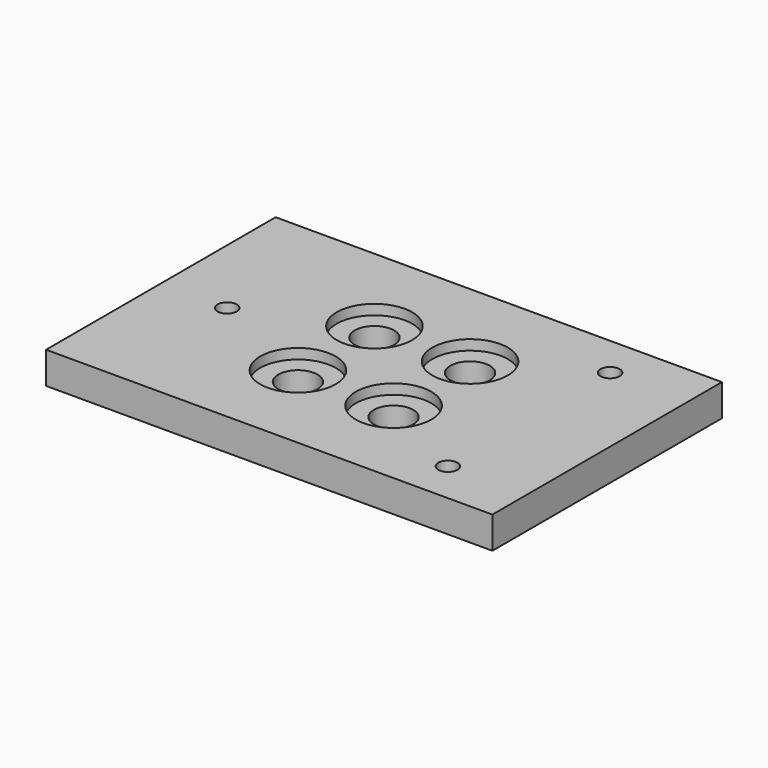
from build123d import *

# Parameters (mm, degrees)
F1_W     = 70
F1_H     = 45
F2_DEPTH = 5
F3_R     = 1.508
F4_DEPTH = 25
F5_R     = 3.0876875
F6_DEPTH = 25
F7_R     = 5.921375
F8_DEPTH = 1.5875


# Not quite as in the source:
# - a length typed as a fraction of an inch, garbled in the dataset ("3 / 203.2 mm" for 3/8 in), is restored


with BuildPart() as f2:
    # F1 (on Top) → F2 (new body)
    with BuildSketch(Plane.XY):
        with Locations((-0.7, 0)):
            Rectangle(F1_W, F1_H)
    extrude(amount=-F2_DEPTH)

    # F3 (on Top) → F4 (cut)
    with BuildSketch(Plane.XY):
        with Locations((-25.3, 0)):
            Circle(F3_R)
        with Locations((22.04, 15.9)):
            Circle(F3_R)
        with Locations((22.04, -15.9)):
            Circle(F3_R)
    extrude(amount=-F4_DEPTH, mode=Mode.SUBTRACT)

    # F5 (on Top) → F6 (cut)
    with BuildSketch(Plane.XY):
        with Locations((-8.2, 7.5)):
            Circle(F5_R)
        with Locations((6.8, 7.5)):
            Circle(F5_R)
        with Locations((-8.2, -7.5)):
            Circle(F5_R)
        with Locations((6.8, -7.5)):
            Circle(F5_R)
    extrude(amount=-F6_DEPTH, mode=Mode.SUBTRACT)

    # F7 (on face) → F8 (cut)
    with BuildSketch(Plane.XY):
        with Locations((-8.2, 7.5)):
            Circle(F7_R)
        with Locations((6.8, 7.5)):
            Circle(F7_R)
        with Locations((-8.2, -7.5)):
            Circle(F7_R)
        with Locations((6.8, -7.5)):
            Circle(F7_R)
    extrude(amount=-F8_DEPTH, mode=Mode.SUBTRACT)


solid = f2.part
